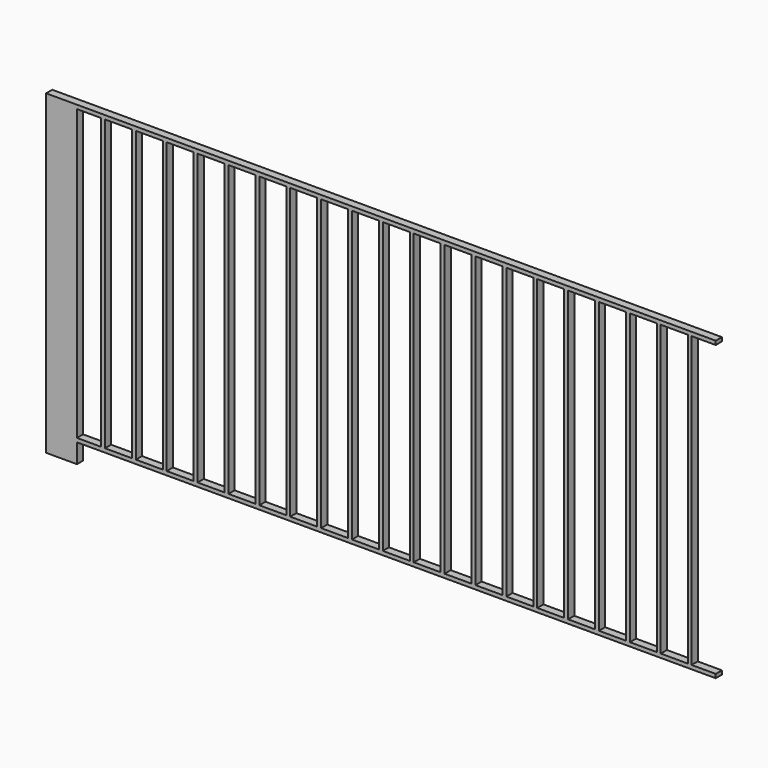
from build123d import *

# Parameters (mm, degrees)
F0_W     = 12.7
F0_H     = 952.5
F1_DEPTH = 25.4


# Not quite as in the source:
# - a feature names something its author has since deleted; it is built from what else it names


with BuildPart() as f1:
    # F0 (on Front) → F1 (new body)
    with BuildSketch(Plane.XZ):
        Polygon((0, 1041.4), (0, 0), (101.6, 0), (101.6, 63.5), (101.6, 76.2), (101.6, 1028.7), (101.6, 1041.4), align=None)
        Polygon((101.6, 76.2), (101.6, 63.5), (2203.45, 63.5), (2203.45, 76.2), (2124.075, 76.2), (2111.375, 76.2), (2022.475, 76.2), (2009.775, 76.2), (1920.875, 76.2), (1908.175, 76.2), (1819.275, 76.2), (1806.575, 76.2), (1717.675, 76.2), (1704.975, 76.2), (1616.075, 76.2), (1603.375, 76.2), (1514.475, 76.2), (1501.775, 76.2), (1412.875, 76.2), (1400.175, 76.2), (1311.275, 76.2), (1298.575, 76.2), (1209.675, 76.2), (1196.975, 76.2), (1108.075, 76.2), (1095.375, 76.2), (1006.475, 76.2), (993.775, 76.2), (904.875, 76.2), (892.175, 76.2), (803.275, 76.2), (790.575, 76.2), (701.675, 76.2), (688.975, 76.2), (600.075, 76.2), (587.375, 76.2), (498.475, 76.2), (485.775, 76.2), (396.875, 76.2), (384.175, 76.2), (295.275, 76.2), (282.575, 76.2), (193.675, 76.2), (180.975, 76.2), align=None)
        with Locations((187.325, 552.45)):
            Rectangle(F0_W, F0_H)
        with Locations((288.925, 552.45)):
            Rectangle(F0_W, F0_H)
        with Locations((390.525, 552.45)):
            Rectangle(F0_W, F0_H)
        with Locations((492.125, 552.45)):
            Rectangle(F0_W, F0_H)
        with Locations((593.725, 552.45)):
            Rectangle(F0_W, F0_H)
        with Locations((695.325, 552.45)):
            Rectangle(F0_W, F0_H)
        with Locations((796.925, 552.45)):
            Rectangle(F0_W, F0_H)
        with Locations((898.525, 552.45)):
            Rectangle(F0_W, F0_H)
        with Locations((1000.125, 552.45)):
            Rectangle(F0_W, F0_H)
        with Locations((1101.725, 552.45)):
            Rectangle(F0_W, F0_H)
        with Locations((1203.325, 552.45)):
            Rectangle(F0_W, F0_H)
        with Locations((1304.925, 552.45)):
            Rectangle(F0_W, F0_H)
        with Locations((1406.525, 552.45)):
            Rectangle(F0_W, F0_H)
        with Locations((1508.125, 552.45)):
            Rectangle(F0_W, F0_H)
        with Locations((1609.725, 552.45)):
            Rectangle(F0_W, F0_H)
        with Locations((1711.325, 552.45)):
            Rectangle(F0_W, F0_H)
        with Locations((1812.925, 552.45)):
            Rectangle(F0_W, F0_H)
        with Locations((1914.525, 552.45)):
            Rectangle(F0_W, F0_H)
        Polygon((2203.45, 1041.4), (101.6, 1041.4), (101.6, 1028.7), (180.975, 1028.7), (193.675, 1028.7), (282.575, 1028.7), (295.275, 1028.7), (384.175, 1028.7), (396.875, 1028.7), (485.775, 1028.7), (498.475, 1028.7), (587.375, 1028.7), (600.075, 1028.7), (688.975, 1028.7), (701.675, 1028.7), (790.575, 1028.7), (803.275, 1028.7), (892.175, 1028.7), (904.875, 1028.7), (993.775, 1028.7), (1006.475, 1028.7), (1095.375, 1028.7), (1108.075, 1028.7), (1196.975, 1028.7), (1209.675, 1028.7), (1298.575, 1028.7), (1311.275, 1028.7), (1400.175, 1028.7), (1412.875, 1028.7), (1501.775, 1028.7), (1514.475, 1028.7), (1603.375, 1028.7), (1616.075, 1028.7), (1704.975, 1028.7), (1717.675, 1028.7), (1806.575, 1028.7), (1819.275, 1028.7), (1908.175, 1028.7), (1920.875, 1028.7), (2009.775, 1028.7), (2022.475, 1028.7), (2111.375, 1028.7), (2124.075, 1028.7), (2203.45, 1028.7), align=None)
        with Locations((2016.125, 552.45)):
            Rectangle(F0_W, F0_H)
        with Locations((2117.725, 552.45)):
            Rectangle(F0_W, F0_H)
    extrude(amount=F1_DEPTH)


solid = f1.part
